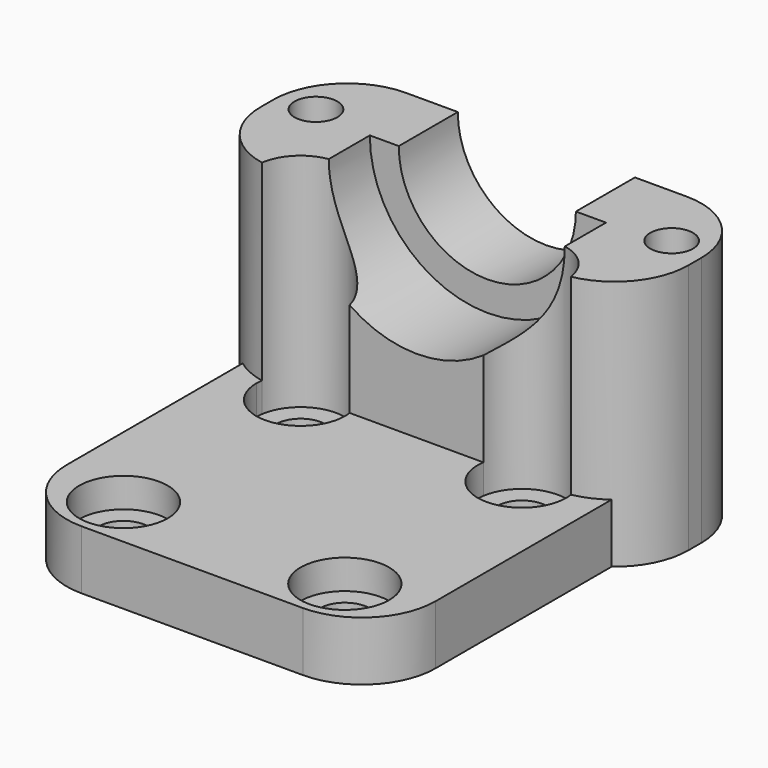
from build123d import *

# Parameters (mm, degrees)
F0_W           = 25
F0_H           = 30
F1_DEPTH       = 4
F2_W           = 25
F2_H           = 11
F3_DEPTH       = 13
F4_R           = 1.675
F5_DEPTH       = 25
F5_DEPTH_BACK  = 25
F7_DEPTH       = 6
F8_R           = 8
F9_DEPTH       = 6
F4_R_2         = 3
F10_DEPTH      = 2
F10_DEPTH_BACK = 25
F11_R          = 5
F13_DEPTH      = 2
F14_W          = 11
F14_H          = 17
F15_DEPTH      = 2
F16_R          = 1.45
F17_DEPTH      = 25
F18_T1_DEPTH   = 42
F18_T6_DEPTH   = 41.5273716251
F18_T11_DEPTH  = 41.5273716251
F18_T16_DEPTH  = 41.5273716251
F18_T21_DEPTH  = 41.5273716251


# Not quite as in the source:
# - a fillet or chamfer that OpenCascade refuses, or shapes differently, is made with other operations: its cross-section is extruded or revolved along the edge and cut away or added


with BuildPart() as f1:
    # F0 (on Top) → F1 (new body)
    with BuildSketch(Plane.XY):
        with Locations((12.5, 15)):
            Rectangle(F0_W, F0_H)
    extrude(amount=F1_DEPTH)

    # F2 (on face) → F3 (join)
    with BuildSketch(Plane.XY.offset(4)):
        with Locations((12.5, 24.5)):
            Rectangle(F2_W, F2_H)
    extrude(amount=F3_DEPTH)

    # F4 (on face) → F5 (cut, two sides)
    with BuildSketch(Plane.XY.offset(4)) as f5_sk:
        with BuildLine():
            ThreePointArc((3.325, 18.5605346784), (5, 16.8855346784), (6.675, 18.5605346784))
            ThreePointArc((6.675, 18.5605346784), (6.6602655711, 18.7822174099), (6.6163215123, 19))
            Line((6.6163215123, 19), (3.3836784877, 19))
            ThreePointArc((3.3836784877, 19), (3.3397344289, 18.7822174099), (3.325, 18.5605346784))
        make_face()
        with BuildLine():
            ThreePointArc((21.6163215123, 19), (20, 20.2355346784), (18.3836784877, 19))
            Line((18.3836784877, 19), (21.6163215123, 19))
        make_face()
        with BuildLine():
            Line((21.6163215123, 19), (18.3836784877, 19))
            ThreePointArc((18.3836784877, 19), (19.7783172685, 16.9002691073), (21.675, 18.5605346784))
            ThreePointArc((21.675, 18.5605346784), (21.6602655711, 18.7822174099), (21.6163215123, 19))
        make_face()
        with Locations((20, 3.5605346784)):
            Circle(F4_R)
        with Locations((5, 3.5605346784)):
            Circle(F4_R)
        with BuildLine():
            Line((3.3836784877, 19), (6.6163215123, 19))
            ThreePointArc((6.6163215123, 19), (5, 20.2355346784), (3.3836784877, 19))
        make_face()
    extrude(amount=-F5_DEPTH, mode=Mode.SUBTRACT)
    extrude(f5_sk.sketch, amount=F5_DEPTH_BACK, mode=Mode.SUBTRACT)

    # F6 (on face) → F7 (cut)
    with BuildSketch(Plane(origin=(0, 30, 0), x_dir=(-1, 0, 0), z_dir=(0, 1, 0))):
        with BuildLine():
            ThreePointArc((-18.5, 17), (-12.5, 11), (-6.5, 17))
            Line((-6.5, 17), (-18.5, 17))
        make_face()
    extrude(amount=-F7_DEPTH, mode=Mode.SUBTRACT)

    # F8 (on face) → F9 (cut)
    with BuildSketch(Plane.XZ.offset(-19)):
        with Locations((12.5394891948, 17)):
            Circle(F8_R)
    extrude(amount=-F9_DEPTH, mode=Mode.SUBTRACT)

    # F4 (on face) → F10 (cut, two sides)
    with BuildSketch(Plane.XY.offset(4)) as f10_sk:
        with BuildLine():
            ThreePointArc((3.3836784877, 19), (5, 20.2355346784), (6.6163215123, 19))
            Line((6.6163215123, 19), (7.9676371461, 19))
            ThreePointArc((7.9676371461, 19), (5, 21.5605346784), (2.0323628539, 19))
            Line((2.0323628539, 19), (3.3836784877, 19))
        make_face()
        with BuildLine():
            Line((2, 18.5605346784), (3.325, 18.5605346784))
            ThreePointArc((3.325, 18.5605346784), (3.3397344289, 18.7822174099), (3.3836784877, 19))
            Line((3.3836784877, 19), (2.0323628539, 19))
            ThreePointArc((2.0323628539, 19), (2.0081016529, 18.7808623453), (2, 18.5605346784))
        make_face()
        with BuildLine():
            ThreePointArc((6.6163215123, 19), (6.6602655711, 18.7822174099), (6.675, 18.5605346784))
            ThreePointArc((6.675, 18.5605346784), (5, 16.8855346784), (3.325, 18.5605346784))
            Line((3.325, 18.5605346784), (2, 18.5605346784))
            ThreePointArc((2, 18.5605346784), (5, 15.5605346784), (8, 18.5605346784))
            ThreePointArc((8, 18.5605346784), (7.9918983471, 18.7808623453), (7.9676371461, 19))
            Line((7.9676371461, 19), (6.6163215123, 19))
        make_face()
        with BuildLine():
            ThreePointArc((22.9676371461, 19), (20, 21.5605346784), (17.0323628539, 19))
            Line((17.0323628539, 19), (18.3836784877, 19))
            ThreePointArc((18.3836784877, 19), (20, 20.2355346784), (21.6163215123, 19))
            Line((21.6163215123, 19), (22.9676371461, 19))
        make_face()
        with BuildLine():
            Line((18.3836784877, 19), (17.0323628539, 19))
            ThreePointArc((17.0323628539, 19), (19.7796723331, 15.5686363313), (23, 18.5605346784))
            ThreePointArc((23, 18.5605346784), (22.9918983471, 18.7808623453), (22.9676371461, 19))
            Line((22.9676371461, 19), (21.6163215123, 19))
            ThreePointArc((21.6163215123, 19), (21.6602655711, 18.7822174099), (21.675, 18.5605346784))
            ThreePointArc((21.675, 18.5605346784), (19.7783172685, 16.9002691073), (18.3836784877, 19))
        make_face()
        with Locations((20, 3.5605346784)):
            Circle(F4_R_2)
        with Locations((20, 3.5605346784)):
            Circle(F4_R, mode=Mode.SUBTRACT)
        with Locations((5, 3.5605346784)):
            Circle(F4_R_2)
        with Locations((5, 3.5605346784)):
            Circle(F4_R, mode=Mode.SUBTRACT)
    extrude(amount=-F10_DEPTH, mode=Mode.SUBTRACT)
    extrude(f10_sk.sketch, amount=F10_DEPTH_BACK, mode=Mode.SUBTRACT)

    # F11
    f11_edges = [f1.edges().sort_by_distance(p)[0] for p in [
        (0, 0, 2),
        (25, 0, 2),
    ]]
    fillet(f11_edges, radius=F11_R)

    # F12 (on face) → F13 (join)
    with BuildSketch(Plane(origin=(0, 0, 0), x_dir=(0, -1, 0), z_dir=(-1, 0, 0))):
        Polygon((-30, 17), (-30, 0), (-19, 0), (-19, 4), (-19, 17), align=None)
    extrude(amount=F13_DEPTH)

    # F14 (on face) → F15 (join)
    with BuildSketch(Plane.YZ.offset(25)):
        with Locations((24.5, 8.5)):
            Rectangle(F14_W, F14_H)
    extrude(amount=F15_DEPTH)

    # F16 (on face) → F17 (cut)
    with BuildSketch(Plane.XY.offset(17)):
        with Locations((0.45, 25.55)):
            Circle(F16_R)
        with Locations((24.55, 25.55)):
            Circle(F16_R)
    extrude(amount=-F17_DEPTH, mode=Mode.SUBTRACT)

    # F18: fillet of radius 5 on 4 edges, made by hand

    # F18_s2 → F18_t1 (cut)
    with BuildSketch(Plane.XY.offset(-12.5)):
        with BuildLine():
            ThreePointArc((-2, 25), (-0.5355339059, 28.5355339059), (3, 30))
            Line((3, 30), (-2, 30))
            Line((-2, 30), (-2, 25))
        make_face()
        with BuildLine():
            ThreePointArc((22, 30), (25.5355339059, 28.5355339059), (27, 25))
            Line((27, 25), (27, 30))
            Line((27, 30), (22, 30))
        make_face()
    extrude(amount=F18_T1_DEPTH, mode=Mode.SUBTRACT)


with BuildPart() as f18_tool4:
    # F18_s5 → F18_t6 (new body)
    with BuildSketch(Plane.XY.offset(29.2636858126)):
        with BuildLine():
            ThreePointArc((2.0323628539, 19), (-0.8625241572, 20.7304298947), (-2, 23.905474325))
            Line((-2, 23.905474325), (-2, 19))
            Line((-2, 19), (2.0323628539, 19))
        make_face()
    extrude(amount=-F18_T6_DEPTH)

    split(bisect_by=Plane.XY.offset(4), keep=Keep.TOP)


with BuildPart() as f1_1:
    add(f1.part)

    # F18_t3: cut F18_tool4
    add(f18_tool4.part, mode=Mode.SUBTRACT)


with BuildPart() as f18_tool9:
    # F18_s10 → F18_t11 (new body)
    with BuildSketch(Plane.XY.offset(29.2636858126)):
        with BuildLine():
            ThreePointArc((2.0323628539, 19), (-0.8625241572, 20.7304298947), (-2, 23.905474325))
            Line((-2, 23.905474325), (-2, 19))
            Line((-2, 19), (2.0323628539, 19))
        make_face()
    extrude(amount=-F18_T11_DEPTH)

    split(bisect_by=Plane.YZ, keep=Keep.BOTTOM)


with BuildPart() as f1_2:
    add(f1_1.part)

    # F18_t8: cut F18_tool9
    add(f18_tool9.part, mode=Mode.SUBTRACT)


with BuildPart() as f18_tool14:
    # F18_s15 → F18_t16 (new body)
    with BuildSketch(Plane.XY.offset(29.2636858126)):
        with BuildLine():
            ThreePointArc((22.9676371461, 19), (25.8625241572, 20.7304298947), (27, 23.905474325))
            Line((27, 23.905474325), (27, 19))
            Line((27, 19), (22.9676371461, 19))
        make_face()
    extrude(amount=-F18_T16_DEPTH)

    split(bisect_by=Plane.XY.offset(4), keep=Keep.TOP)


with BuildPart() as f1_3:
    add(f1_2.part)

    # F18_t13: cut F18_tool14
    add(f18_tool14.part, mode=Mode.SUBTRACT)


with BuildPart() as f18_tool19:
    # F18_s20 → F18_t21 (new body)
    with BuildSketch(Plane.XY.offset(29.2636858126)):
        with BuildLine():
            ThreePointArc((22.9676371461, 19), (25.8625241572, 20.7304298947), (27, 23.905474325))
            Line((27, 23.905474325), (27, 19))
            Line((27, 19), (22.9676371461, 19))
        make_face()
    extrude(amount=-F18_T21_DEPTH)

    split(bisect_by=Plane.YZ.offset(25), keep=Keep.TOP)


with BuildPart() as f1_4:
    add(f1_3.part)

    # F18_t18: cut F18_tool19
    add(f18_tool19.part, mode=Mode.SUBTRACT)


solid = f1_4.part
